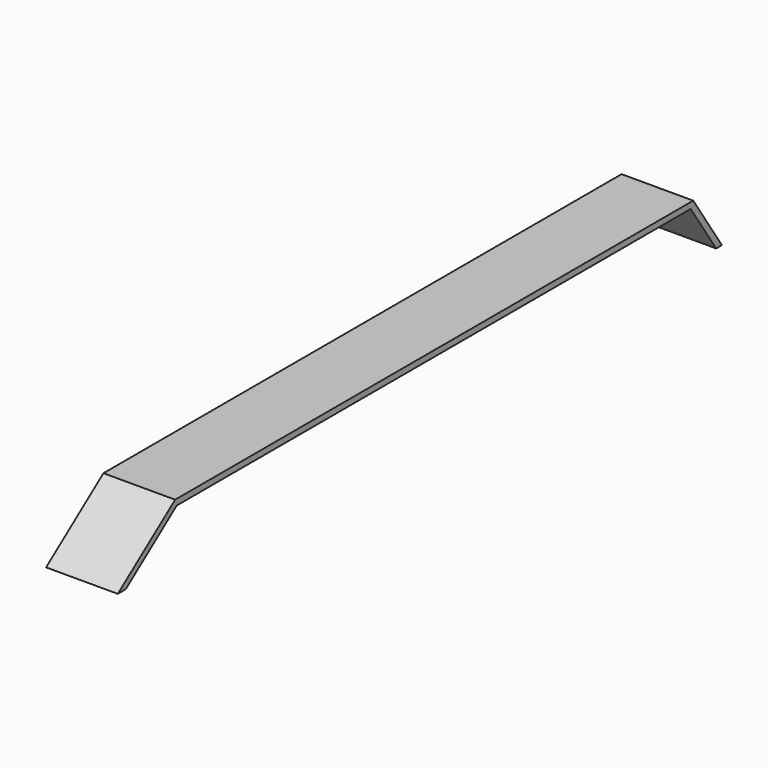
from build123d import *

# Parameters (mm, degrees)
F0_W     = 30
F0_H     = 316
F1_DEPTH = 5
F2_DEPTH = 17.5
F3_SIZE2 = 14.99999
F3_SIZE  = 22.49999
F4_SIZE2 = 22.49999
F4_SIZE  = 29.99999
F5_T     = 2.5
F6_DEPTH = 2.4
F7_DEPTH = 25


# Not quite as in the source:
# - a fillet or chamfer is up to 0.001 mm smaller than in the source, because OpenCascade refuses the exact size
# - a shell that OpenCascade refuses in one call is made with other operations: the cavity is built on its own and cut out


with BuildPart() as f1:
    # F0 (on Top) → F1 (new body)
    with BuildSketch(Plane.XY):
        Rectangle(F0_W, F0_H)
    extrude(amount=F1_DEPTH)

    # F2 (add): a face of the model
    f2_faces = [f1.faces().sort_by_distance(p)[0] for p in [
        (0, 0, 0),
    ]]
    extrude(f2_faces, amount=F2_DEPTH)

    # F3 (size 22.5 and 15 in the source; OpenCascade refuses exactly that, so slightly less here)
    f3_edges = [f1.edges().sort_by_distance(p)[0] for p in [
        (0, 158, 5),
    ]]
    f3_side = f1.faces().sort_by_distance((0, 158, -6.25))[0]
    chamfer(f3_edges, length=F3_SIZE, length2=F3_SIZE2, reference=f3_side)

    # F4 (size 30 and 22.5 in the source; OpenCascade refuses exactly that, so slightly less here)
    f4_edges = [f1.edges().sort_by_distance(p)[0] for p in [
        (0, -158, 5),
    ]]
    f4_side = f1.faces().sort_by_distance((0, -7.499995, 5))[0]
    chamfer(f4_edges, length=F4_SIZE, length2=F4_SIZE2, reference=f4_side)

    # F5: shell of thickness 2.5, made by hand


with BuildPart() as f5_core1:
    # F5_t2: copy of F1
    add(f1.part)

    # the walls: a layer under each face that stays
    f5_faces = [f5_core1.faces().sort_by_distance(p)[0] for p in [
        (15, 0, -6.25),
        (0, 7.5, 5),
        (0, -143.000005, -6.249995),
        (0, 150.500005, -6.249995),
        (0, -158, -17.499995),
        (0, 158, -17.499995),
        (-15, 0, -6.25),
    ]]
    thicken(f5_faces, amount=-F5_T, mode=Mode.SUBTRACT)


with BuildPart() as f1_1:
    add(f1.part)

    # what is left inside the walls is the cavity
    f5_cavity = [f5_core1.part.solids().sort_by_distance(p)[0] for p in [
        (0, -50.890437, -17.475),
    ]]
    add(f5_cavity, mode=Mode.SUBTRACT)

    # F6 (cut): a face of the model
    f6_faces = [f1_1.faces().sort_by_distance(p)[0] for p in [
        (-12.5, 3.8374129004, -7.7308172989),
    ]]
    extrude(f6_faces, amount=-F6_DEPTH, mode=Mode.SUBTRACT)

    # F7 (cut): a face of the model
    f7_faces = [f1_1.faces().sort_by_distance(p)[0] for p in [
        (12.5, 3.8374129004, -7.7308172989),
    ]]
    extrude(f7_faces, amount=-F7_DEPTH, mode=Mode.SUBTRACT)


solid = f1_1.part
